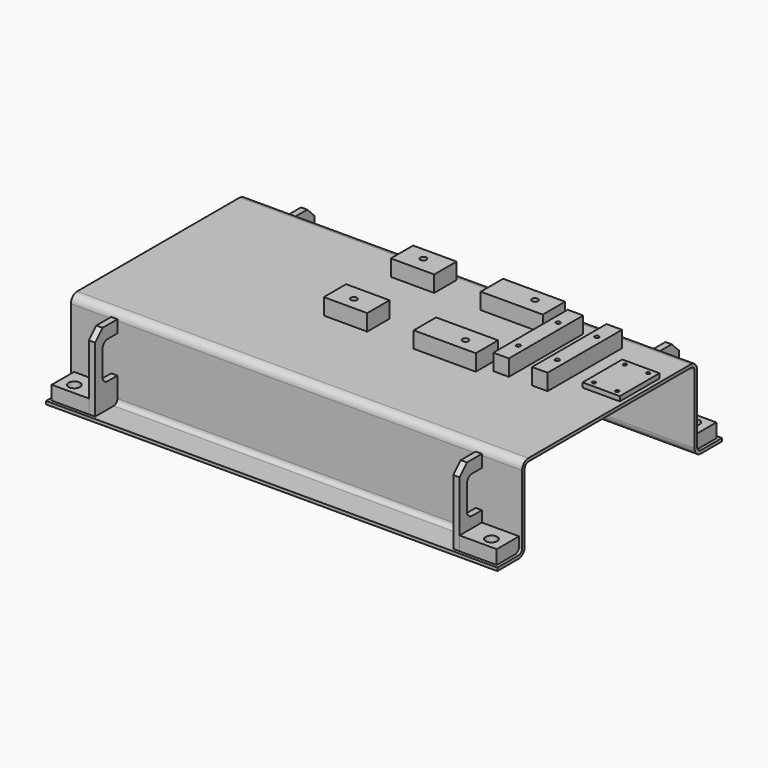
from build123d import *

# Parameters (mm, degrees)
F1_DEPTH  = 923.925
F2_W      = 152.4
F2_H      = 114.3
F2_R      = 23.8125
F3_DEPTH  = 57.15
F5_DEPTH  = 25.4
F6_SIZE   = 38.1
F9_W      = 152.4
F9_H      = 203.2
F10_DEPTH = 19.05
F12_D     = 14.2875
F14_DEPTH = 66.548
F16_D     = 17.4625
F17_W     = 177.8
F17_H     = 114.3
F17_W_2   = 254
F18_DEPTH = 66.675
F20_D     = 25.4


# Not quite as in the source:
# - a length typed as a fraction of an inch, garbled in the dataset ("3 / 203.2 mm" for 3/8 in), is restored


with BuildPart() as f1:
    # F0 (on Right) → F1 (new body, symmetric)
    with BuildSketch(Plane.YZ):
        with BuildLine():
            Line((0, 171.45), (-415.925, 171.45))
            ThreePointArc((-415.925, 171.45), (-438.3756403027, 162.1506403027), (-447.675, 139.7))
            Line((-447.675, 139.7), (-447.675, -139.7))
            ThreePointArc((-447.675, -139.7), (-453.2546158184, -153.1703841816), (-466.725, -158.75))
            Line((-466.725, -158.75), (-574.675, -158.75))
            Line((-574.675, -158.75), (-574.675, -171.45))
            Line((-574.675, -171.45), (-466.725, -171.45))
            ThreePointArc((-466.725, -171.45), (-444.2743596973, -162.1506403027), (-434.975, -139.7))
            Line((-434.975, -139.7), (-434.975, 139.7))
            ThreePointArc((-434.975, 139.7), (-429.3953841816, 153.1703841816), (-415.925, 158.75))
            Line((-415.925, 158.75), (0, 158.75))
            Line((0, 158.75), (415.925, 158.75))
            ThreePointArc((415.925, 158.75), (429.3953841816, 153.1703841816), (434.975, 139.7))
            Line((434.975, 139.7), (434.975, -139.7))
            ThreePointArc((434.975, -139.7), (444.2743596973, -162.1506403027), (466.725, -171.45))
            Line((466.725, -171.45), (574.675, -171.45))
            Line((574.675, -171.45), (574.675, -158.75))
            Line((574.675, -158.75), (466.725, -158.75))
            ThreePointArc((466.725, -158.75), (453.2546158184, -153.1703841816), (447.675, -139.7))
            Line((447.675, -139.7), (447.675, 139.7))
            ThreePointArc((447.675, 139.7), (438.3756403027, 162.1506403027), (415.925, 171.45))
            Line((415.925, 171.45), (0, 171.45))
        make_face()
    extrude(amount=F1_DEPTH, both=True)

    # F9 (on face) → F10 (join)
    with BuildSketch(Plane.XY.offset(171.45)):
        with Locations((830.961, 174.625)):
            Rectangle(F9_W, F9_H)
    extrude(amount=F10_DEPTH)

    # F12 (through all)
    with Locations(Plane.XY.offset(190.5)):
        with Locations((783.336, 254), (878.586, 254), (783.336, 95.25), (878.586, 95.25)):
            Hole(F12_D / 2)

    # F13 (on face) → F14 (join)
    with BuildSketch(Plane.XY.offset(171.45)):
        Polygon((523.748, 174.625), (523.748, 365.125), (460.248, 365.125), (460.248, 174.625), (460.248, -15.875), (523.748, -15.875), align=None)
        Polygon((682.498, 365.125), (618.998, 365.125), (618.998, 174.625), (618.998, -15.875), (682.498, -15.875), (682.498, 174.625), align=None)
    extrude(amount=F14_DEPTH)

    # F16 (through all)
    with Locations(Plane.XY.offset(237.998)):
        with Locations((491.998, 276.225), (650.748, 276.225), (491.998, 73.025), (650.748, 73.025)):
            Hole(F16_D / 2)

    # F17 (on face) → F18 (join)
    with BuildSketch(Plane.XY.offset(171.45)):
        with Locations((-114.427, 3.175)):
            Rectangle(F17_W, F17_H)
        with Locations((-114.427, 346.075)):
            Rectangle(F17_W, F17_H)
        with Locations((291.973, 346.075)):
            Rectangle(F17_W_2, F17_H)
        with Locations((291.973, 3.175)):
            Rectangle(F17_W_2, F17_H)
    extrude(amount=F18_DEPTH)

    # F20 (through all)
    with Locations(Plane.XY.offset(238.125)):
        with Locations((-120.777, 352.425), (336.423, 352.425), (-120.777, -3.175), (336.423, -3.175)):
            Hole(F20_D / 2)


with BuildPart() as f3:
    # F2 (on face) → F3 (new body)
    with BuildSketch(Plane.XY.offset(-158.75)):
        with Locations((835.025, -504.825)):
            Rectangle(F2_W, F2_H)
        with Locations((854.075, -517.525)):
            Circle(F2_R, mode=Mode.SUBTRACT)
    extrude(amount=F3_DEPTH)


with BuildPart() as f5:
    # F4 (on face) → F5 (new body)
    with BuildSketch(Plane(origin=(758.825, 0, 0), x_dir=(0, -1, 0), z_dir=(-1, 0, 0))):
        with BuildLine():
            Line((447.675, -57.15), (447.675, -158.75))
            Line((447.675, -158.75), (561.975, -158.75))
            Line((561.975, -158.75), (561.975, 146.05))
            Line((561.975, 146.05), (447.675, 146.05))
            Line((447.675, 146.05), (447.675, 95.25))
            Line((447.675, 95.25), (498.475, 95.25))
            ThreePointArc((498.475, 95.25), (516.4355122421, 87.8105122421), (523.875, 69.85))
            Line((523.875, 69.85), (523.875, -31.75))
            ThreePointArc((523.875, -31.75), (516.4355122421, -49.7105122421), (498.475, -57.15))
            Line((498.475, -57.15), (447.675, -57.15))
        make_face()
    extrude(amount=F5_DEPTH)

    # F6
    f6_edges = [f5.edges().sort_by_distance(p)[0] for p in [
        (746.125, -561.975, 146.05),
    ]]
    chamfer(f6_edges, length=F6_SIZE)


with BuildPart() as f7_1:
    # F7: instance of F5
    add(f5.part.mirror(Plane.YZ))


with BuildPart() as f7_2:
    # F7: instance of F3
    add(f3.part.mirror(Plane.YZ))


with BuildPart() as f8_1:
    # F8: instance of F3
    add(f3.part.mirror(Plane.XZ))


with BuildPart() as f8_2:
    # F8: instance of F5
    add(f5.part.mirror(Plane.XZ))


with BuildPart() as f8_3:
    # F8: instance of F7_2
    add(f7_2.part.mirror(Plane.XZ))


with BuildPart() as f8_4:
    # F8: instance of F7_1
    add(f7_1.part.mirror(Plane.XZ))


solid = Compound([f1.part, f3.part, f5.part, f7_1.part, f7_2.part, f8_1.part, f8_2.part, f8_3.part, f8_4.part])
